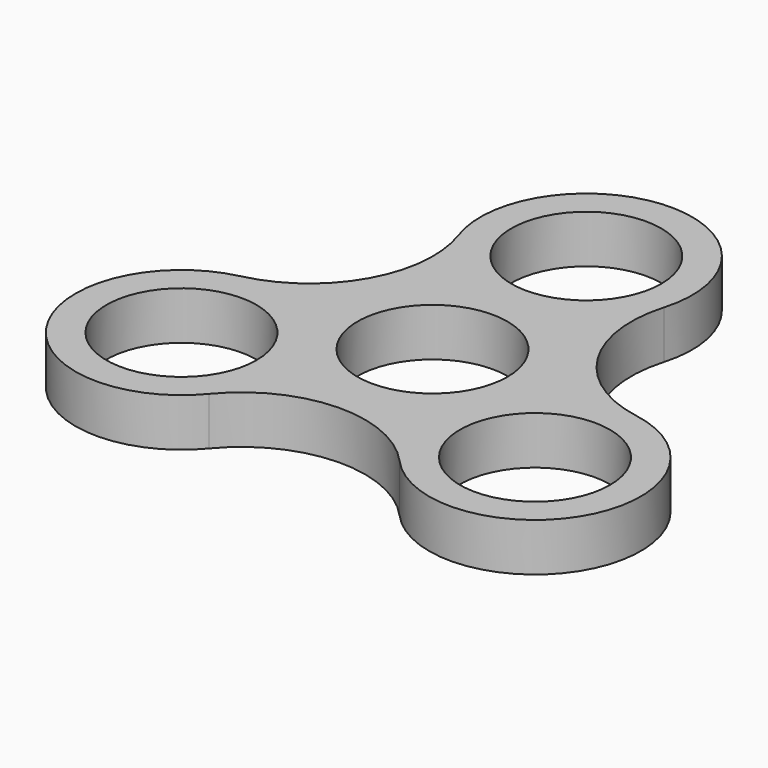
from build123d import *

# Parameters (mm, degrees)
F0_R     = 10.92
F1_DEPTH = 7


# Not quite as in the source:
# - a feature names something its author has since deleted; it is built from what else it names


with BuildPart() as f1:
    # F0 (on Top) → F1 (new body)
    with BuildSketch(Plane.XY):
        with BuildLine():
            ThreePointArc((28.3529823071, 1.6761283467), (16.1276038689, 9.8932258121), (14.1316130419, 24.4876284834))
            ThreePointArc((14.1316130419, 24.4876284834), (-1.0184797386, 44.2482801815), (-15.2433325814, 23.8114940253))
            ThreePointArc((-15.2433325814, 23.8114940253), (-16.5331807129, 9.1989312159), (-28.2699008548, 0.3989255129))
            ThreePointArc((-28.2699008548, 0.3989255129), (-37.9772339165, -22.7266382845), (-12.9562617696, -24.4514481107))
            ThreePointArc((-12.9562617696, -24.4514481107), (0.5300904983, -17.9124126397), (14.291675769, -23.8503797349))
            ThreePointArc((14.291675769, -23.8503797349), (39.2470886778, -20.9610002997), (28.3529823071, 1.6761283467))
        make_face()
        with Locations((-24.849640726, -14.6369722206)):
            Circle(F0_R, mode=Mode.SUBTRACT)
        Circle(F0_R, mode=Mode.SUBTRACT)
        with Locations((25.7406966372, -13.5209886029)):
            Circle(F0_R, mode=Mode.SUBTRACT)
        with Locations((-0.6636456317, 28.8323633176)):
            Circle(F0_R, mode=Mode.SUBTRACT)
    extrude(amount=F1_DEPTH)


solid = f1.part
